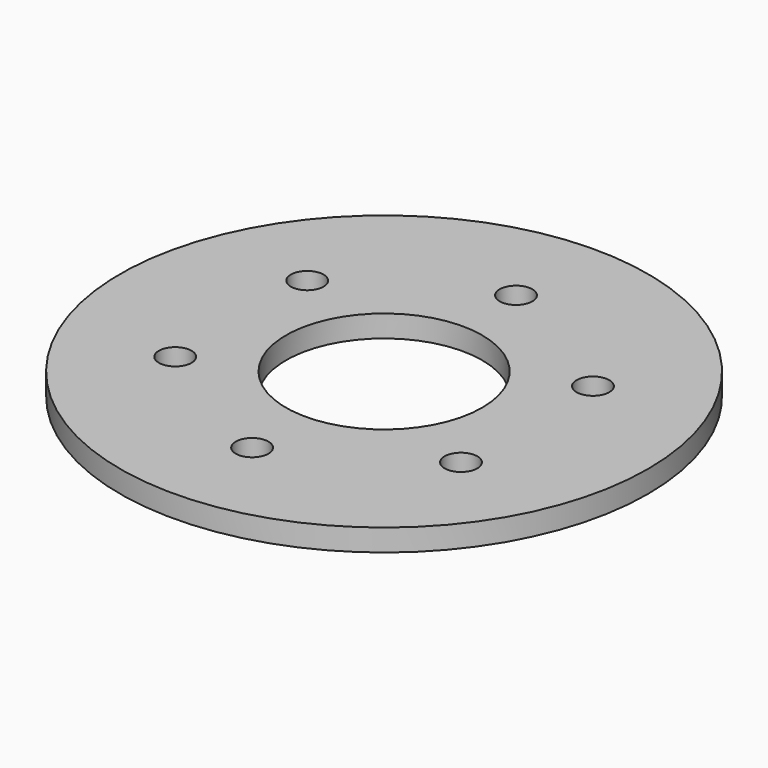
from build123d import *

# Parameters (mm, degrees)
F0_R            = 38.1
F0_R_2          = 14.1605
F1_DEPTH        = 3.175
F2_R            = 2.3622
F3_DEPTH        = 3.176
F3_COPIES_COUNT = 6


# Not quite as in the source:
# - a pattern or mirror of a feature is missing from the dataset's text; its kind, count and spacing are read off the source's solid


with BuildPart() as f1:
    # F0 (on Top) → F1 (new body)
    with BuildSketch(Plane.XY):
        Circle(F0_R)
        Circle(F0_R_2, mode=Mode.SUBTRACT)
    extrude(amount=F1_DEPTH)

    # F2 (on face) → F3 (cut, through all)
    with BuildSketch(Plane.XY.offset(3.175)):
        with Locations((0, 23.8125)):
            Circle(F2_R)
    f3 = extrude(amount=-F3_DEPTH, mode=Mode.SUBTRACT)

    # F3_copies: F3 ×6 about axis
    f3_copies_axis = Axis((0, 0, 0), (0, 0, 1))
    for i in range(1, F3_COPIES_COUNT):
        add(f3.rotate(f3_copies_axis, i * 360 / F3_COPIES_COUNT), mode=Mode.SUBTRACT)


solid = f1.part
